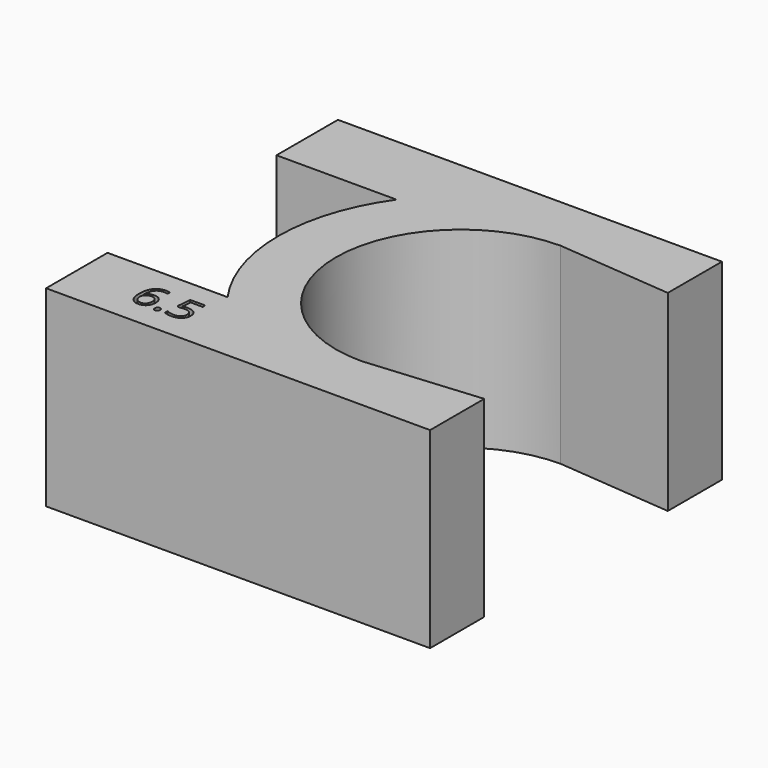
from build123d import *

# Parameters (mm, degrees)
F1_DEPTH     = 5
F2_TEXT_SIZE = 1.1034906586
F3_DEPTH     = 2


# Not quite as in the source:
# - Text() gives the source's letters only with a copy of the font that has no kerning and outlines rounded to 1/6400 em; it was checked with that copy


with BuildPart() as f1:
    # F0 (on Top) → F1 (new body)
    with BuildSketch(Plane.XY):
        with BuildLine():
            ThreePointArc((0, -3.25), (-3.25, 0), (0, 3.25))
            Line((0, 3.25), (3, 2.9875340094))
            Line((3, 2.9875340094), (3, 4.75))
            Line((3, 4.75), (0, 4.75))
            Line((0, 4.75), (-7, 4.75))
            Line((-7, 4.75), (-7, 2.75))
            Line((-7, 2.75), (-3.8729833462, 2.75))
            ThreePointArc((-3.8729833462, 2.75), (-4.75, 0), (-3.8729833462, -2.75))
            Line((-3.8729833462, -2.75), (-7, -2.75))
            Line((-7, -2.75), (-7, -4.75))
            Line((-7, -4.75), (0, -4.75))
            Line((0, -4.75), (3, -4.75))
            Line((3, -4.75), (3, -2.9875340094))
            Line((3, -2.9875340094), (0, -3.25))
        make_face()
    extrude(amount=F1_DEPTH)

    # F2 (on face) → F3 (cut)
    with BuildSketch(Plane.XY.offset(5)):
        with Locations((-5.4364916731, -4.1078054757)):
            Text('6.5', F2_TEXT_SIZE, font='Open Sans', text_align=(TextAlign.LEFT, TextAlign.BOTTOM))
    extrude(amount=-F3_DEPTH, mode=Mode.SUBTRACT)


solid = f1.part
